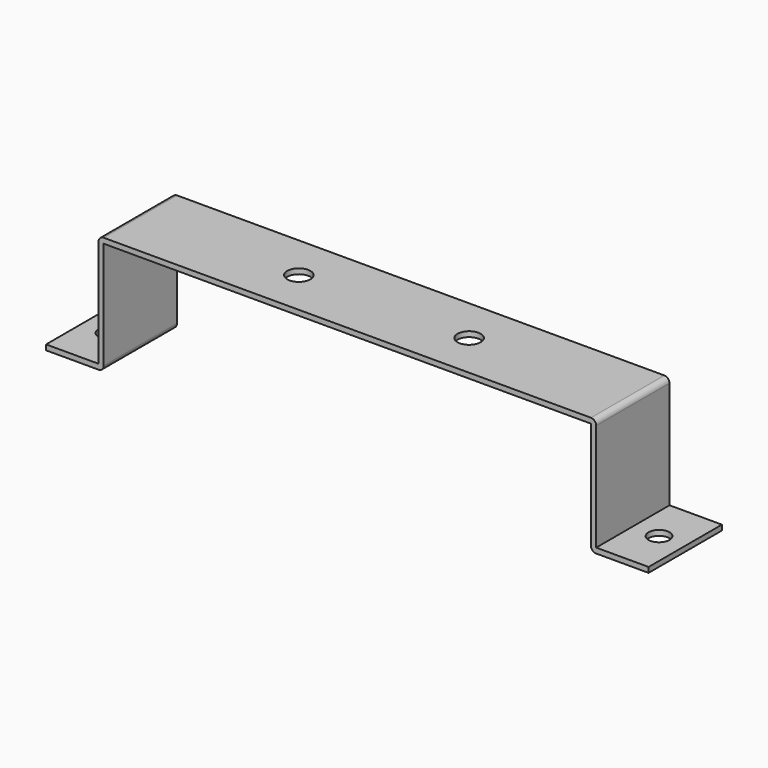
from build123d import *

# Parameters (mm, degrees)
F1_DEPTH = 17.5
F2_R     = 4
F3_DEPTH = 25
F4_R     = 4.4
F5_DEPTH = 25
F6_R     = 2


# Not quite as in the source:
# - a feature names something its author has since deleted; it is built from what else it names


with BuildPart() as f1:
    # F0 (on Front) → F1 (new body, symmetric)
    with BuildSketch(Plane.XZ):
        Polygon((95, -38), (95, 5), (-95, 5), (-95, -38), (-115, -38), (-115, -40), (-93, -40), (-93, 3), (93, 3), (93, -40), (115, -40), (115, -38), align=None)
    extrude(amount=F1_DEPTH, both=True)

    # F2 (on face) → F3 (cut)
    with BuildSketch(Plane.XY.offset(-38)):
        with Locations((-105, 0)):
            Circle(F2_R)
        with Locations((105, 0)):
            Circle(F2_R)
    extrude(amount=-F3_DEPTH, mode=Mode.SUBTRACT)

    # F4 (on face) → F5 (cut)
    with BuildSketch(Plane.XY.offset(5)):
        with Locations((-32.5, 0)):
            Circle(F4_R)
        with Locations((32.5, 0)):
            Circle(F4_R)
    extrude(amount=-F5_DEPTH, mode=Mode.SUBTRACT)

    # F6
    f6_edges = [f1.edges().sort_by_distance(p)[0] for p in [
        (95, 0, 5),
        (-95, 0, 5),
        (-93, 0, -40),
        (93, 0, -40),
    ]]
    fillet(f6_edges, radius=F6_R)


solid = f1.part
